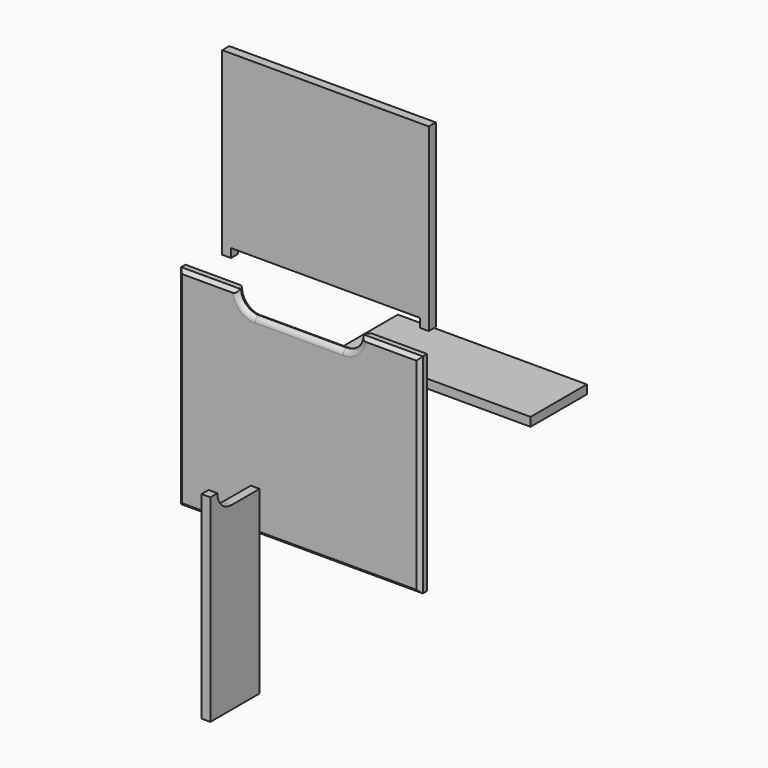
from build123d import *

# Parameters (mm, degrees)
F1_DEPTH     = 12.7
F2_SIZE      = 5.08
F3_T3_DEPTH  = 127
F3_T6_DEPTH  = 127
F3_T9_ANGLE  = 132.9890967712
F3_T12_ANGLE = 132.9890967712
F3_T15_ANGLE = 121.447994897
F3_T18_ANGLE = 121.447994897
F4_W         = 273.05
F4_H         = 101.6
F5_DEPTH     = 12.7
F7_DEPTH     = 12.7
F9_DEPTH     = 12.7


# Not quite as in the source:
# - a fillet or chamfer that OpenCascade refuses, or shapes differently, is made with other operations: its cross-section is extruded or revolved along the edge and cut away or added


with BuildPart() as f1:
    # F0 (on Front) → F1 (new body)
    with BuildSketch(Plane.XZ):
        with BuildLine():
            Line((-97.1290172577, 136.0299303359), (-182.8540172577, 136.0299303359))
            Line((-182.8540172577, 136.0299303359), (-182.8540172577, -165.5950696641))
            Line((-182.8540172577, -165.5950696641), (166.3959827423, -165.5950696641))
            Line((166.3959827423, -165.5950696641), (166.3959827423, 136.0299303359))
            Line((166.3959827423, 136.0299303359), (80.6709827423, 136.0299303359))
            ThreePointArc((80.6709827423, 136.0299303359), (73.2314949844, 118.0694180937), (55.2709827423, 110.6299303359))
            Line((55.2709827423, 110.6299303359), (-71.7290172577, 110.6299303359))
            ThreePointArc((-71.7290172577, 110.6299303359), (-89.6895294998, 118.0694180937), (-97.1290172577, 136.0299303359))
        make_face()
    extrude(amount=F1_DEPTH)

    # F2
    f2_edges = [f1.edges().sort_by_distance(p)[0] for p in [
        (-8.229017, -12.7, -165.59507),
        (166.395983, -12.7, -14.78257),
        (-182.854017, -12.7, -14.78257),
        (-139.991517, -12.7, 136.02993),
        (123.533483, -12.7, 136.02993),
    ]]
    chamfer(f2_edges, length=F2_SIZE)

    # F3: fillet of radius 7.62 on 2 edges, made by hand


with BuildPart() as f3_tool1:
    # F3_s2 → F3_t3 (new body)
    with BuildSketch(Plane.YZ.offset(55.2709827423)):
        with BuildLine():
            ThreePointArc((-12.7, 103.0099303359), (-10.4681536726, 108.3980840085), (-5.08, 110.6299303359))
            Line((-5.08, 110.6299303359), (-12.7, 110.6299303359))
            Line((-12.7, 110.6299303359), (-12.7, 103.0099303359))
        make_face()
    extrude(amount=-F3_T3_DEPTH)


with BuildPart() as f3_tool4:
    # F3_s5 → F3_t6 (new body)
    with BuildSketch(Plane.YZ.offset(55.2709827423)):
        with BuildLine():
            ThreePointArc((0, 103.0099303359), (-2.2318463274, 108.3980840085), (-7.62, 110.6299303359))
            Line((-7.62, 110.6299303359), (0, 110.6299303359))
            Line((0, 110.6299303359), (0, 103.0099303359))
        make_face()
    extrude(amount=-F3_T6_DEPTH)


with BuildPart() as f3_tool7:
    # F3_s8 → F3_t9 (revolve)
    with BuildSketch(Plane(origin=(-42.1502287044, 0, 45.217835005), x_dir=(0, 1, 0), z_dir=(-0.6818591731, 0, 0.7314834708))):
        with BuildLine():
            ThreePointArc((0, -166.2030661087), (-2.2318463274, -160.8149124361), (-7.62, -158.5830661087))
            Line((-7.62, -158.5830661087), (0, -158.5830661087))
            Line((0, -158.5830661087), (0, -166.2030661087))
        make_face()
    revolve(axis=Axis((55.2709827423, 0, 136.0299303359), (0, 1, 0)), revolution_arc=F3_T9_ANGLE)


with BuildPart() as f3_tool10:
    # F3_s11 → F3_t12 (revolve)
    with BuildSketch(Plane.YZ.offset(-71.7290172577)):
        with BuildLine():
            ThreePointArc((-7.62, 110.6299303359), (-2.2318463274, 108.3980840085), (0, 103.0099303359))
            Line((0, 103.0099303359), (0, 110.6299303359))
            Line((0, 110.6299303359), (-7.62, 110.6299303359))
        make_face()
    revolve(axis=Axis((-71.7290172577, 0, 136.0299303359), (0, 1, 0)), revolution_arc=F3_T12_ANGLE)


with BuildPart() as f3_tool13:
    # F3_s14 → F3_t15 (revolve)
    with BuildSketch(Plane(origin=(-45.5010619878, 0, 74.4024868236), x_dir=(0, 1, 0), z_dir=(-0.521724442, 0, 0.8531140643))):
        with BuildLine():
            ThreePointArc((-12.7, -151.1425922207), (-10.4681536726, -145.7544385481), (-5.08, -143.5225922207))
            Line((-5.08, -143.5225922207), (-12.7, -143.5225922207))
            Line((-12.7, -143.5225922207), (-12.7, -151.1425922207))
        make_face()
    revolve(axis=Axis((55.2709827423, -12.7, 136.0299303359), (0, 1, 0)), revolution_arc=F3_T15_ANGLE)


with BuildPart() as f3_tool16:
    # F3_s17 → F3_t18 (revolve)
    with BuildSketch(Plane.YZ.offset(-71.7290172577)):
        with BuildLine():
            ThreePointArc((-5.08, 110.6299303359), (-10.4681536726, 108.3980840085), (-12.7, 103.0099303359))
            Line((-12.7, 103.0099303359), (-12.7, 110.6299303359))
            Line((-12.7, 110.6299303359), (-5.08, 110.6299303359))
        make_face()
    revolve(axis=Axis((-71.7290172577, -12.7, 136.0299303359), (0, 1, 0)), revolution_arc=F3_T18_ANGLE)


with BuildPart() as f1_1:
    add(f1.part)

    # F3_t19: cut F3_tool1, F3_tool4, F3_tool7, F3_tool10, F3_tool13, F3_tool16
    add([f3_tool1.part, f3_tool4.part, f3_tool7.part, f3_tool10.part, f3_tool13.part, f3_tool16.part], mode=Mode.SUBTRACT)


with BuildPart() as f5:
    # F4 (on Top) → F5 (new body)
    with BuildSketch(Plane.XY):
        with Locations((69.1801686266, 188.6979788542)):
            Rectangle(F4_W, F4_H)
    extrude(amount=F5_DEPTH)


with BuildPart() as f7:
    # F6 (on Right) → F7 (new body)
    with BuildSketch(Plane.YZ):
        with BuildLine():
            ThreePointArc((-161.1934086972, -40.7115346551), (-179.1539209393, -33.2720468972), (-186.5934086972, -15.3115346551))
            Line((-186.5934086972, -15.3115346551), (-199.2934086972, -15.3115346551))
            Line((-199.2934086972, -15.3115346551), (-199.2934086972, -301.0615346551))
            Line((-199.2934086972, -301.0615346551), (-110.3934086972, -301.0615346551))
            Line((-110.3934086972, -301.0615346551), (-110.3934086972, -40.7115346551))
            Line((-110.3934086972, -40.7115346551), (-161.1934086972, -40.7115346551))
        make_face()
    extrude(amount=F7_DEPTH)


with BuildPart() as f9:
    # F8 (on face) → F9 (new body)
    with BuildSketch(Plane.XZ.offset(12.7)):
        Polygon((189.165537107, 443.1593230724), (-109.284462893, 443.1593230724), (-109.284462893, 195.5093230724), (-109.284462893, 182.8093230724), (-96.584462893, 182.8093230724), (-96.584462893, 195.5093230724), (176.465537107, 195.5093230724), (176.465537107, 182.8093230724), (189.165537107, 182.8093230724), (189.165537107, 195.5093230724), align=None)
    extrude(amount=F9_DEPTH)


solid = Compound([f1_1.part, f5.part, f7.part, f9.part])
